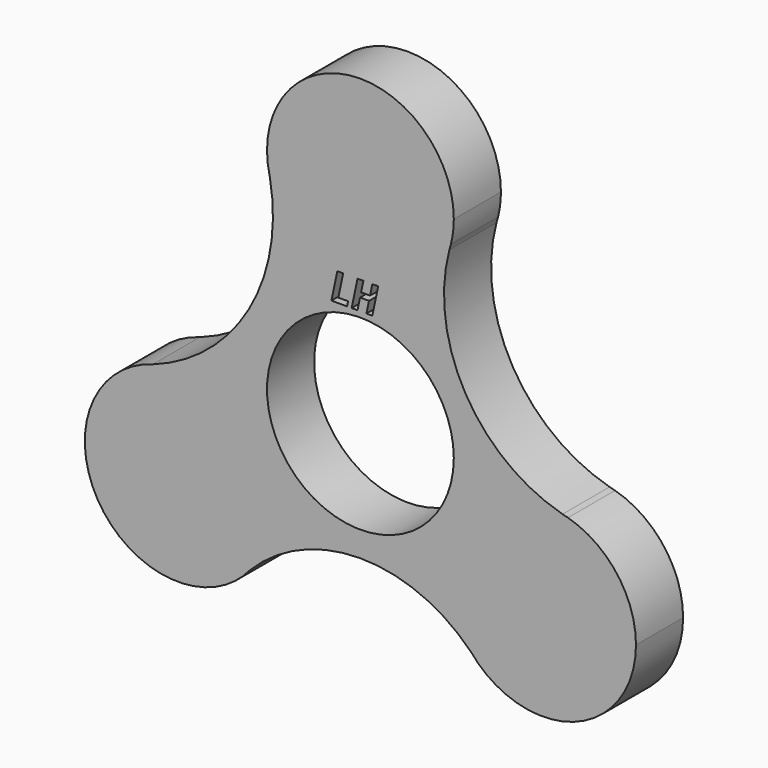
from build123d import *

# Parameters (mm, degrees)
F0_R         = 11.1
F1_DEPTH     = 7
F2_TEXT_SIZE = 4.6347009225
F3_DEPTH     = 12.7


# Not quite as in the source:
# - Text() gives the source's letters only with a copy of the font that has no kerning and outlines rounded to 1/6400 em; it was checked with that copy


with BuildPart() as f1:
    # F0 (on Front) → F1 (new body)
    with BuildSketch(Plane.XZ):
        with BuildLine():
            ThreePointArc((10.5768459141, 21.6324592788), (-0.3340251326, 13.9050269396), (-10.7602728632, 22.2748343338))
            ThreePointArc((-10.7602728632, 22.2748343338), (-13.2609230977, 7.6561975202), (-24.6707088297, -1.8187475157))
            ThreePointArc((-24.6707088297, -1.8187475157), (-14.9540993656, -3.6475196001), (-10.5506350946, -12.5))
            ThreePointArc((-10.5506350946, -12.5), (-11.2049874754, -16.2547897164), (-13.0908956017, -19.5668847319))
            ThreePointArc((-13.0908956017, -19.5668847319), (0, -14.0843518452), (13.0908956017, -19.5668847319))
            ThreePointArc((13.0908956017, -19.5668847319), (12.176030139, -6.7171061799), (24.0226822388, -1.6564123859))
            ThreePointArc((24.0226822388, -1.6564123859), (12.4846792181, 7.2080329073), (10.5768459141, 21.6324592788))
        make_face()
        Circle(F0_R, mode=Mode.SUBTRACT)
        with BuildLine():
            ThreePointArc((-10.5506350946, -12.5), (-14.9540993656, -3.6475196001), (-24.6707088297, -1.8187475157))
            ThreePointArc((-24.6707088297, -1.8187475157), (-31.2635170766, -18.05), (-13.9104359665, -20.4560868181))
            ThreePointArc((-13.9104359665, -20.4560868181), (-13.5079845537, -20.0047403713), (-13.0908956017, -19.5668847319))
            ThreePointArc((-13.0908956017, -19.5668847319), (-11.2049874754, -16.2547897164), (-10.5506350946, -12.5))
        make_face()
        with BuildLine():
            ThreePointArc((24.6707088297, -1.8187475157), (24.3459834367, -1.7404225776), (24.0226822388, -1.6564123859))
            ThreePointArc((24.0226822388, -1.6564123859), (12.176030139, -6.7171061799), (13.0908956017, -19.5668847319))
            ThreePointArc((13.0908956017, -19.5668847319), (13.5079845537, -20.0047403713), (13.9104359665, -20.4560868181))
            ThreePointArc((13.9104359665, -20.4560868181), (25.9688401429, -22.7256102586), (32.7506350946, -12.5))
            ThreePointArc((32.7506350946, -12.5), (30.5031154945, -5.803464271), (24.6707088297, -1.8187475157))
        make_face()
        with BuildLine():
            ThreePointArc((10.7602728632, 22.2748343338), (11.0147407773, 23.6268701413), (11.1, 25))
            ThreePointArc((11.1, 25), (-1.3731298587, 36.0147407773), (-10.7602728632, 22.2748343338))
            ThreePointArc((-10.7602728632, 22.2748343338), (-0.3340251326, 13.9050269396), (10.5768459141, 21.6324592788))
            ThreePointArc((10.5768459141, 21.6324592788), (10.6657415528, 21.9544514251), (10.7602728632, 22.2748343338))
        make_face()
    extrude(amount=F1_DEPTH)

    # F2 (on face) → F3 (cut)
    with BuildSketch(Plane.XZ.offset(7)):
        with Locations((-3.5587195307, 11.7511479184)):
            Text('LH', F2_TEXT_SIZE, font='Open Sans', font_style=FontStyle.BOLDITALIC, text_align=(TextAlign.LEFT, TextAlign.BOTTOM))
    extrude(amount=-F3_DEPTH, mode=Mode.SUBTRACT)


solid = f1.part
